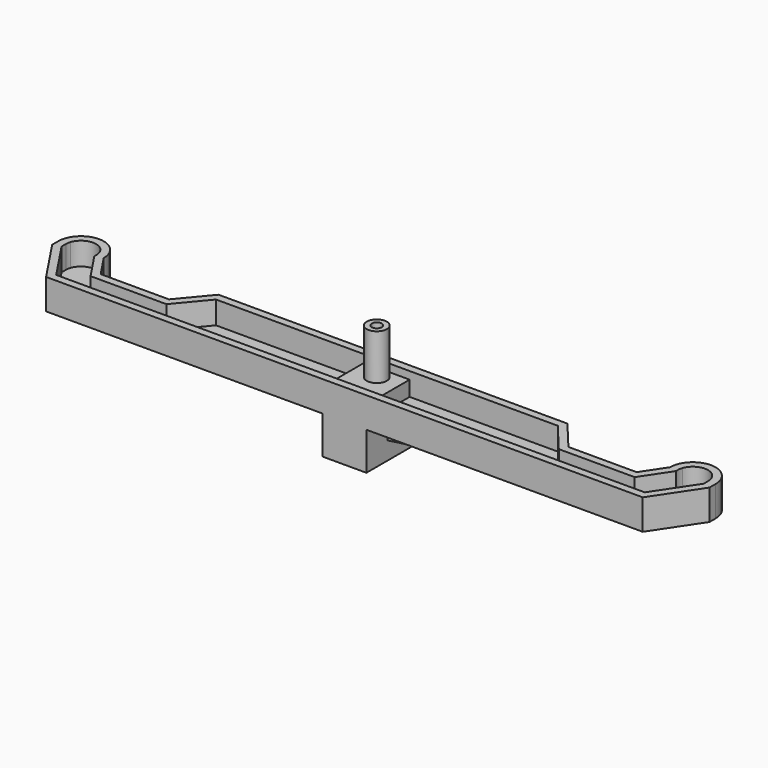
from build123d import *

# Parameters (mm, degrees)
F1_DEPTH  = 6
F3_T      = -1.5
F4_R      = 1
F5_DEPTH  = 26
F6_W      = 9
F6_H      = 9
F7_DEPTH  = 3
F8_R      = 2
F8_R_2    = 1
F9_DEPTH  = 9
F11_DEPTH = 7.5
F12_DEPTH = 2.5
F14_DEPTH = 0.75


# Not quite as in the source:
# - a feature names something its author has since deleted; it is built from what else it names


with BuildPart() as f1:
    # F0 (on Top) → F1 (new body)
    with BuildSketch(Plane.XY):
        with BuildLine():
            Line((-65, 4.5), (-65, 3))
            Line((-65, 3), (-59, -6))
            Line((-59, -6), (0, -6))
            Line((0, -6), (0, 6))
            Line((0, 6), (-34.5, 6))
            Line((-34.5, 6), (-39.5, 0))
            Line((-39.5, 0), (-53, 0))
            Line((-53, 0), (-56, 4.5))
            ThreePointArc((-56, 4.5), (-60.5, 0), (-65, 4.5))
        make_face()
        with BuildLine():
            ThreePointArc((-64.7426406871, 6), (-64.9351935184, 5.2609589043), (-65, 4.5))
            ThreePointArc((-65, 4.5), (-60.5, 0), (-56, 4.5))
            ThreePointArc((-56, 4.5), (-56.0648064816, 5.2609589043), (-56.2573593129, 6))
            Line((-56.2573593129, 6), (-64.7426406871, 6))
        make_face()
        with BuildLine():
            ThreePointArc((-56.2573593129, 6), (-60.5, 9), (-64.7426406871, 6))
            Line((-64.7426406871, 6), (-56.2573593129, 6))
        make_face()
    extrude(amount=F1_DEPTH)

    # F2: F1 across plane


with BuildPart() as f1_1:
    add(f1.part)
    add(f1.part.mirror(Plane.YZ))

    # F3
    f3_openings = [f1_1.faces().sort_by_distance(p)[0] for p in [
        (0, -0.200074, 6),
    ]]
    offset(amount=F3_T, openings=f3_openings, kind=Kind.INTERSECTION)

    # F4 (on face) → F5 (cut)
    with BuildSketch(Plane.XY.offset(1.5)):
        with BuildLine():
            ThreePointArc((-57.5283708886, 4.0883928763), (-57.5071011265, 4.2937081366), (-57.5, 4.5))
            ThreePointArc((-57.5, 4.5), (-60.5, 7.5), (-63.5, 4.5))
            ThreePointArc((-63.5, 4.5), (-60.7062918634, 1.5071011265), (-57.5283708886, 4.0883928763))
        make_face()
        with Locations((-60.5, 4.5)):
            Circle(F4_R, mode=Mode.SUBTRACT)
    extrude(amount=F5_DEPTH, mode=Mode.SUBTRACT)

    # F6 (on face) → F7 (join)
    with BuildSketch(Plane.XY.offset(1.5)):
        Rectangle(F6_W, F6_H)
    extrude(amount=F7_DEPTH)

    # F8 (on face) → F9 (join)
    with BuildSketch(Plane.XY.offset(4.5)):
        with Locations((0, 2)):
            Circle(F8_R)
        with Locations((0, 2)):
            Circle(F8_R_2, mode=Mode.SUBTRACT)
    extrude(amount=F9_DEPTH)

    # F10 (on face) → F11 (join)
    with BuildSketch(Plane(origin=(0, 0, 0), x_dir=(1, 0, 0), z_dir=(0, 0, -1))):
        Polygon((4.35, 6), (-4.35, 6), (-4.35, -6), (-2.85, -6), (-2.85, 4.5), (2.85, 4.5), (2.85, -6), (4.35, -6), align=None)
    extrude(amount=F11_DEPTH)

    # F12 (cut): a face of the model
    f12_faces = [f1_1.faces().sort_by_distance(p)[0] for p in [
        (0, 0.75, 0),
    ]]
    extrude(f12_faces, amount=-F12_DEPTH, mode=Mode.SUBTRACT)

    # F13 (on Front) → F14 (join, symmetric)
    with BuildSketch(Plane.XZ):
        Polygon((4.35, 0), (4.35, -4), (14.85, -2.5), (14.85, 0), align=None)
        Polygon((-14.85, -2.5), (-4.35, -4), (-4.35, 0), (-14.85, 0), align=None)
    extrude(amount=F14_DEPTH, both=True)


solid = f1_1.part
